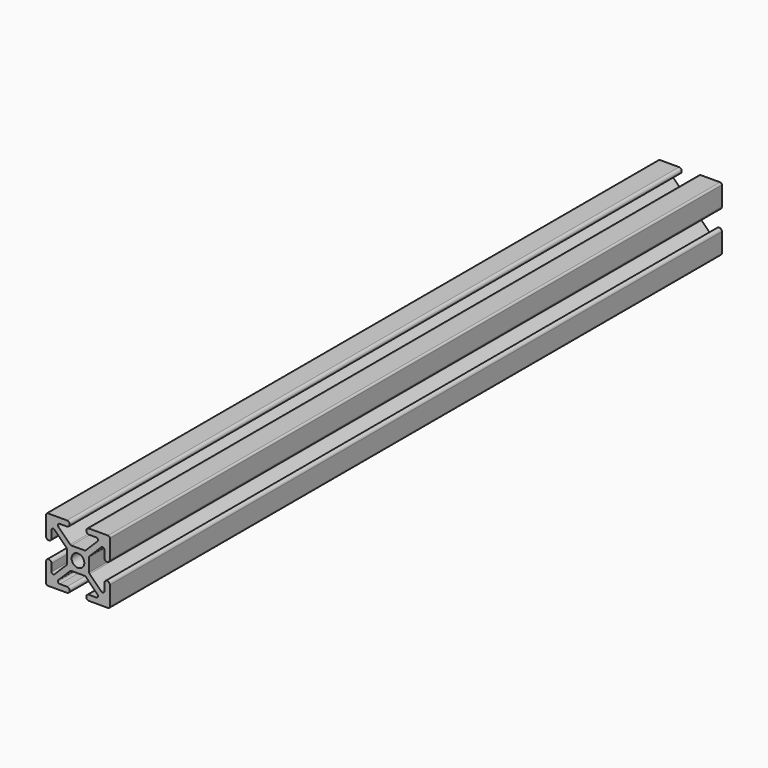
from build123d import *

# Parameters (mm, degrees)
F0_R     = 2.5
F1_DEPTH = 300


# Not quite as in the source:
# - ends of sketch curves that miss each other by under 0.0002 mm in the source are joined


with BuildPart() as f1:
    # F0 (on Front) → F1 (new body)
    with BuildSketch(Plane.XZ):
        with BuildLine():
            ThreePointArc((12.5, 11.8), (12.2949747468, 12.2949747468), (11.8, 12.5))
            Line((11.8, 12.5), (4.3149960966, 12.5))
            ThreePointArc((4.3149960966, 12.5), (3.5629475094, 12.1890874766), (3.25, 11.4378834224))
            Line((3.25, 11.4378834224), (3.2499960966, 11.4350005532))
            ThreePointArc((3.2499960966, 11.4350005532), (3.5619271791, 10.6819314736), (4.3149960966, 10.37))
            Line((4.3149960966, 10.37), (7.1739130624, 10.37))
            ThreePointArc((7.1739130624, 10.37), (7.8206287352, 9.9378784027), (7.6688878092, 9.1750252532))
            Line((7.6688878092, 9.1750252532), (3.0788878092, 4.5850252532))
            ThreePointArc((3.0788878092, 4.5850252532), (2.8517914651, 4.4332843272), (2.5839130624, 4.38))
            Line((2.5839130624, 4.38), (-2.5839130624, 4.38))
            ThreePointArc((-2.5839130624, 4.38), (-2.8517914651, 4.4332843272), (-3.0788878092, 4.5850252532))
            Line((-3.0788878092, 4.5850252532), (-7.6688878092, 9.1750252532))
            ThreePointArc((-7.6688878092, 9.1750252532), (-7.8206287352, 9.9378784027), (-7.1739130624, 10.37))
            Line((-7.1739130624, 10.37), (-4.3149983424, 10.37))
            ThreePointArc((-4.3149983424, 10.37), (-3.2499983424, 11.435), (-4.3149983424, 12.5))
            Line((-4.3149983424, 12.5), (-11.8, 12.5))
            ThreePointArc((-11.8, 12.5), (-12.2949747468, 12.2949747468), (-12.5, 11.8))
            Line((-12.5, 11.8), (-12.5, 4.3148727296))
            ThreePointArc((-12.5, 4.3148727296), (-11.435, 3.2498727296), (-10.37, 4.3148727296))
            Line((-10.37, 4.3148727296), (-10.37, 7.1739130624))
            ThreePointArc((-10.37, 7.1739130624), (-9.9378784027, 7.8206287352), (-9.1750252532, 7.6688878092))
            Line((-9.1750252532, 7.6688878092), (-4.5850252532, 3.0788878092))
            ThreePointArc((-4.5850252532, 3.0788878092), (-4.4332843272, 2.8517914651), (-4.38, 2.5839130624))
            Line((-4.38, 2.5839130624), (-4.38, -2.5839130624))
            ThreePointArc((-4.38, -2.5839130624), (-4.4332843272, -2.8517914651), (-4.5850252532, -3.0788878092))
            Line((-4.5850252532, -3.0788878092), (-9.1750252532, -7.6688878092))
            ThreePointArc((-9.1750252532, -7.6688878092), (-9.9378784027, -7.8206287352), (-10.37, -7.1739130624))
            Line((-10.37, -7.1739130624), (-10.37, -4.3142225218))
            ThreePointArc((-10.37, -4.3142225218), (-11.435, -3.2492225218), (-12.5, -4.3142225218))
            Line((-12.5, -4.3142225218), (-12.5, -11.8))
            ThreePointArc((-12.5, -11.8), (-12.2949747468, -12.2949747468), (-11.8, -12.5))
            Line((-11.8, -12.5), (-4.3149983424, -12.5))
            ThreePointArc((-4.3149983424, -12.5), (-3.2499983424, -11.435), (-4.3149983424, -10.37))
            Line((-4.3149983424, -10.37), (-7.1739130624, -10.37))
            ThreePointArc((-7.1739130624, -10.37), (-7.8206287352, -9.9378784027), (-7.6688878092, -9.1750252532))
            Line((-7.6688878092, -9.1750252532), (-3.0788878092, -4.5850252532))
            ThreePointArc((-3.0788878092, -4.5850252532), (-2.8517914651, -4.4332843272), (-2.5839130624, -4.38))
            Line((-2.5839130624, -4.38), (2.5839130624, -4.38))
            ThreePointArc((2.5839130624, -4.38), (2.8517914651, -4.4332843272), (3.0788878092, -4.5850252532))
            Line((3.0788878092, -4.5850252532), (7.6688878092, -9.1750252532))
            ThreePointArc((7.6688878092, -9.1750252532), (7.8206287352, -9.9378784027), (7.1739130624, -10.37))
            Line((7.1739130624, -10.37), (4.3149960966, -10.37))
            ThreePointArc((4.3149960966, -10.37), (3.2499960966, -11.435), (4.3149960966, -12.5))
            Line((4.3149960966, -12.5), (11.8, -12.5))
            ThreePointArc((11.8, -12.5), (12.2949747468, -12.2949747468), (12.5, -11.8))
            Line((12.5, -11.8), (12.5, -4.3148727296))
            Line((12.5, -4.3148727296), (12.5, -4.3142225218))
            ThreePointArc((12.5, -4.3142225218), (11.435, -3.2498727296), (10.3700001985, -4.314222522))
            Line((10.3700001985, -4.314222522), (10.37, -4.3148727296))
            Line((10.37, -4.3148727296), (10.37, -7.1739130624))
            ThreePointArc((10.37, -7.1739130624), (9.9378784027, -7.8206287352), (9.1750252532, -7.6688878092))
            Line((9.1750252532, -7.6688878092), (4.5850252532, -3.0788878092))
            ThreePointArc((4.5850252532, -3.0788878092), (4.4332843272, -2.8517914651), (4.38, -2.5839130624))
            Line((4.38, -2.5839130624), (4.38, 2.5839130624))
            ThreePointArc((4.38, 2.5839130624), (4.4332843272, 2.8517914651), (4.5850252532, 3.0788878092))
            Line((4.5850252532, 3.0788878092), (9.1750252532, 7.6688878092))
            ThreePointArc((9.1750252532, 7.6688878092), (9.9378784027, 7.8206287352), (10.37, 7.1739130624))
            Line((10.37, 7.1739130624), (10.37, 4.3148727296))
            ThreePointArc((10.37, 4.3148727296), (10.3700000496, 4.3145476258), (10.3700001985, 4.314222522))
            ThreePointArc((10.3700001985, 4.314222522), (11.435, 3.2498727296), (12.4999998015, 4.314222522))
            ThreePointArc((12.4999998015, 4.314222522), (12.4999999504, 4.3145476258), (12.5, 4.3148727296))
            Line((12.5, 4.3148727296), (12.5, 11.8))
        make_face()
        Circle(F0_R, mode=Mode.SUBTRACT)
        with BuildLine():
            ThreePointArc((10.37, 4.3142225218), (11.435, 3.2492225218), (12.5, 4.3142225218))
            ThreePointArc((12.5, 4.3142225218), (11.435, 3.2498727296), (10.37, 4.3142225218))
        make_face()
        with BuildLine():
            ThreePointArc((12.5, -4.3142225218), (11.435, -3.2492225218), (10.37, -4.3142225218))
            ThreePointArc((10.37, -4.3142225218), (11.435, -3.2498727296), (12.5, -4.3142225218))
        make_face()
    extrude(amount=F1_DEPTH)


solid = f1.part
